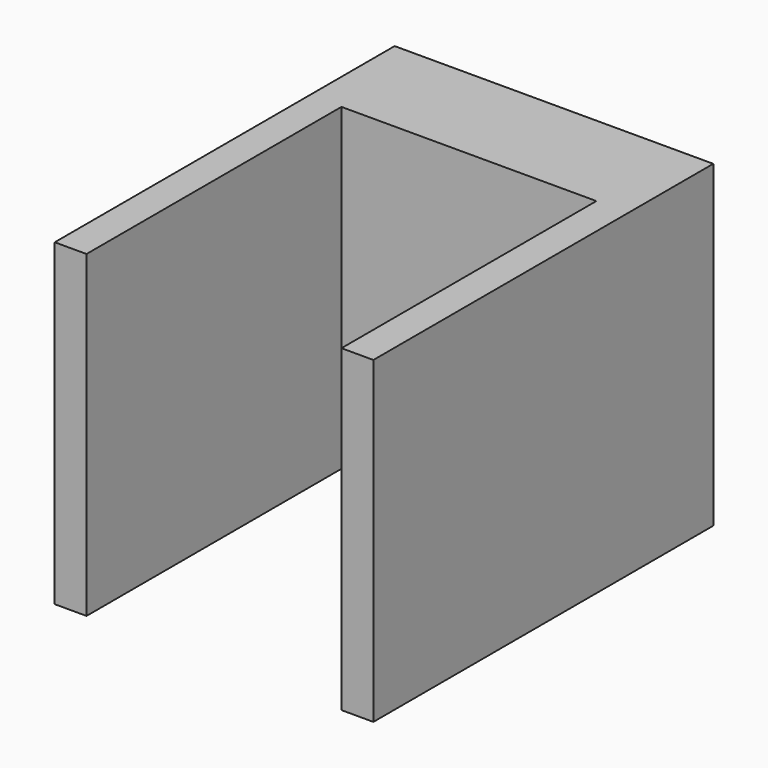
from build123d import *

# Parameters (mm, degrees)
F0_W     = 25.4
F0_H     = 19.05
F1_DEPTH = 9.525
F2_W     = 15.2418981306
F2_H     = 19.05
F3_DEPTH = 19.05


# Not quite as in the source:
# - a feature names something its author has since deleted; it is built from what else it names


with BuildPart() as f1:
    # F0 (on Right) → F1 (new body, symmetric)
    with BuildSketch(Plane.YZ):
        with Locations((-12.7, 9.525)):
            Rectangle(F0_W, F0_H)
    extrude(amount=F1_DEPTH, both=True)

    # F2 (on face) → F3 (cut)
    with BuildSketch(Plane.XZ.offset(25.4)):
        with Locations((-0.004085945, 9.525)):
            Rectangle(F2_W, F2_H)
    extrude(amount=-F3_DEPTH, mode=Mode.SUBTRACT)


solid = f1.part
